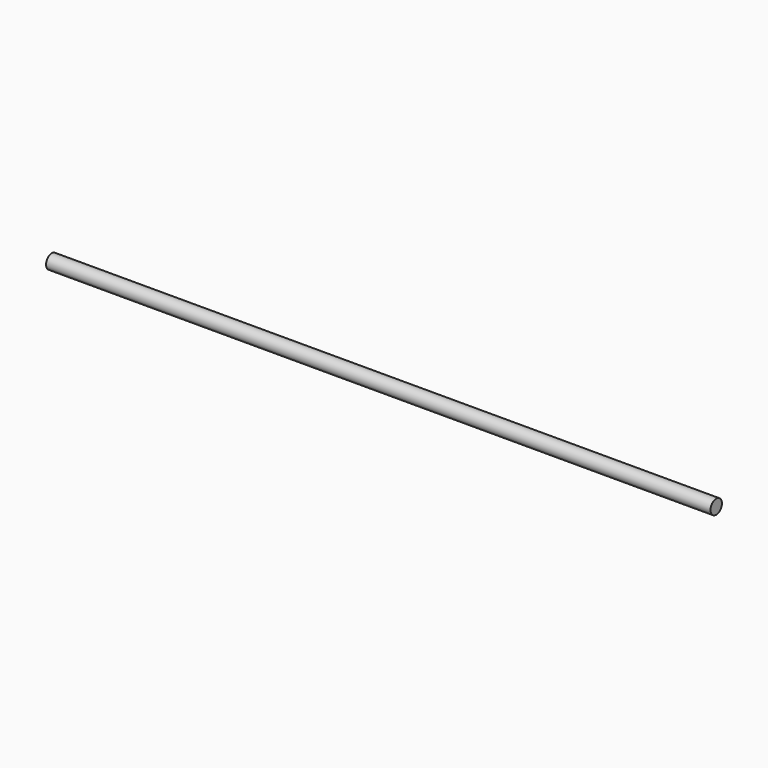
from build123d import *

# Parameters (mm, degrees)
F0_R     = 4.825
F1_DEPTH = 450
F2_D     = 1.5113
F2_DEPTH = 19.690625
F2_TIP   = 0.4540403268


# Not quite as in the source:
# - a feature of the source that left no trace in its solid (it failed there, or was rolled back) is left out


with BuildPart() as f1:
    # F0 (on Right) → F1 (new body)
    with BuildSketch(Plane.YZ):
        Circle(F0_R)
    extrude(amount=F1_DEPTH)

    # F2
    with Locations(Plane(origin=(0, 0, 0), x_dir=(0, 1, 0), z_dir=(-1, 0, 0))):
        with Locations((0, 0), (0, 0), (0, 0)):
            Hole(F2_D / 2, depth=F2_DEPTH)
            with Locations((0, 0, -(F2_DEPTH + F2_TIP / 2))):  # 118° drill point
                Cone(0, F2_D / 2, F2_TIP, mode=Mode.SUBTRACT)


solid = f1.part
